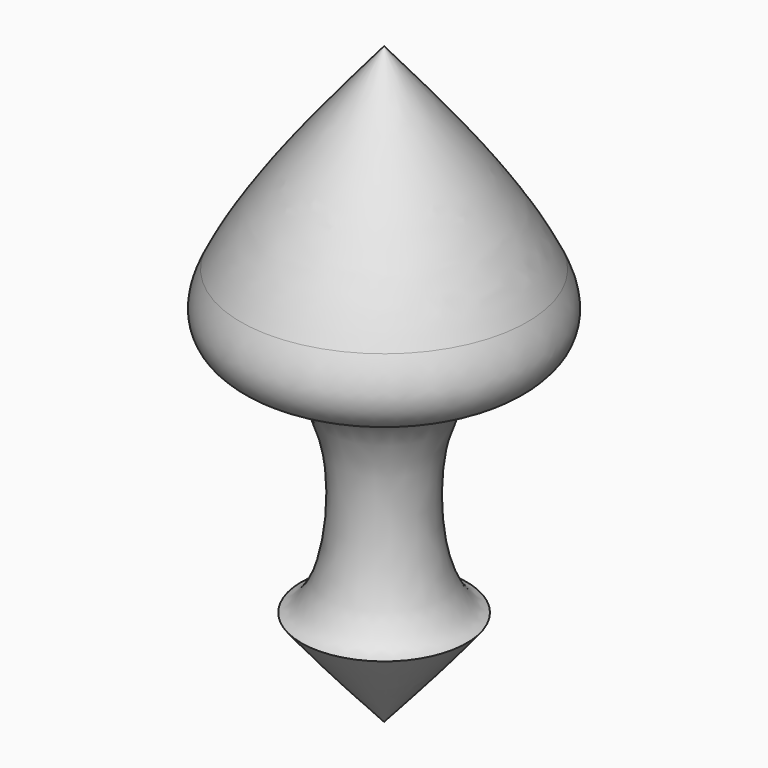
from build123d import *


# Not quite as in the source:
# - a fillet or chamfer that OpenCascade refuses, or shapes differently, is made with other operations: its cross-section is extruded or revolved along the edge and cut away or added


with BuildPart() as f1:
    # F0 (on Front) → F1 (revolve)
    with BuildSketch(Plane.XZ):
        with BuildLine():
            Line((0, 0), (0, 53.0163384974))
            add(Edge.make_bspline(
                [(0, 53.0163384974), (-7.7204488092, 43.8814871891), (-15.4408976031, 34.7466358989), (-15.3417233382, 25.8284714426)],
                knots=[0, 0, 0, 0, 0.5048017032, 0.5048017032, 0.5048017032, 0.5048017032], degree=3))
            add(Edge.make_bspline(
                [(-15.3417233186, 25.8284714568), (-13.9391664267, 29.4549986533), (-1.5172985659, 29.5779810102), (-3.9619687384, 9.400148093), (-7.3695517839, 8.5805750916)],
                knots=[0.3760425959, 0.3760425959, 0.3760425959, 0.3760425959, 0.6398968964, 0.991433205, 0.991433205, 0.991433205, 0.991433205], degree=3))
            add(Edge.make_bspline(
                [(-7.3695517819, 8.5805751172), (-5.1009829868, 5.7151752374), (-2.5504914934, 2.8575876187), (0, 0)],
                knots=[0.8343003226, 0.8343003226, 0.8343003226, 0.8343003226, 1, 1, 1, 1], degree=3))
        make_face()
    revolve(axis=Axis((0, 0, 26.5081692487), (0, 0, -1)))

    # F2: fillet of radius 5.08 on 1 edges, made by hand

    # F2_s1 → F2_t2 (revolve, cut)
    with BuildSketch(Plane.XZ):
        with BuildLine():
            add(Edge.make_bspline(
                [(-12.7770843094, 35.5268361891), (-15.539496918, 29.9919695065), (-9.5731143471, 28.3585829531)],
                knots=[0, 0, 0, 1, 1, 1], degree=2, weights=[1, 1, 1]))
            Line((-9.5731143471, 28.3585829531), (-9.5999417115, 28.2605888078))
            ThreePointArc((-9.5999417115, 28.2605888078), (-12.8599796885, 28.1560554661), (-15.2469633294, 25.7918230855))
            Line((-15.2469633294, 25.7918230855), (-15.4433170468, 25.8273416789))
            ThreePointArc((-15.4433170468, 25.8273416789), (-14.7296425373, 30.8674166322), (-12.8679910731, 35.5722071085))
            Line((-12.8679910731, 35.5722071085), (-12.7770843094, 35.5268361891))
        make_face()
    revolve(axis=Axis((0, 0, 25.8284714497), (0, 0, -1)), mode=Mode.SUBTRACT)


solid = f1.part
